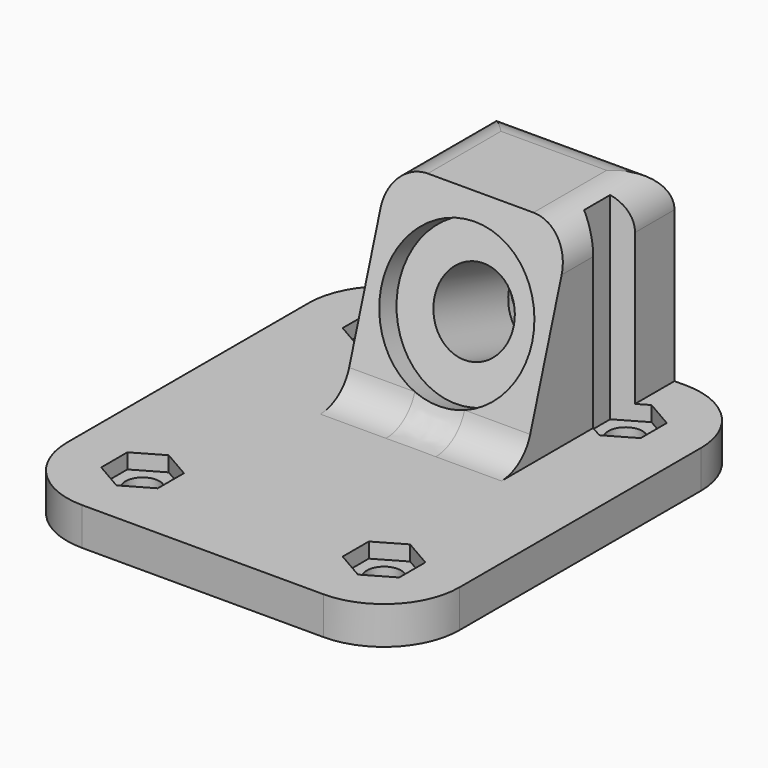
from build123d import *

# Parameters (mm, degrees)
F0_W         = 52
F0_H         = 60
F1_DEPTH     = 5
F2_R         = 10
F3_R         = 2.25
F4_DEPTH     = 25
F6_DEPTH     = 2
F7_W         = 24
F7_H         = 25
F8_DEPTH     = 25
F10_DEPTH    = 35.501
F11_R        = 5.25
F12_DEPTH    = 25.3474527662
F13_R        = 10
F13_R_2      = 5.25
F14_DEPTH    = 3
F16_R        = 10
F17_DEPTH    = 12
F18_DEPTH    = 25.001
F19_F1_R     = 5
F19_T2_DEPTH = 42.117530278
F19_T4_DEPTH = 31.5358983849
F19_T6_DEPTH = 28.6534286629
F19_T8_DEPTH = 49


# Not quite as in the source:
# - a fillet or chamfer that OpenCascade refuses, or shapes differently, is made with other operations: its cross-section is extruded or revolved along the edge and cut away or added


with BuildPart() as f1:
    # F0 (on Top) → F1 (new body)
    with BuildSketch(Plane.XY):
        Rectangle(F0_W, F0_H)
    extrude(amount=F1_DEPTH)

    # F2
    f2_edges = [f1.edges().sort_by_distance(p)[0] for p in [
        (26, -30, 2.5),
        (-26, -30, 2.5),
        (26, 30, 2.5),
        (-26, 30, 2.5),
    ]]
    fillet(f2_edges, radius=F2_R)

    # F3 (on face) → F4 (cut)
    with BuildSketch(Plane.XY.offset(5)):
        with Locations((-16, -20)):
            Circle(F3_R)
        with Locations((16, -20)):
            Circle(F3_R)
        with Locations((-16, 20)):
            Circle(F3_R)
        with Locations((16, 20)):
            Circle(F3_R)
    extrude(amount=-F4_DEPTH, mode=Mode.SUBTRACT)

    # F5 (on face) → F6 (cut)
    with BuildSketch(Plane.XY.offset(5)):
        Polygon((-16, -15.6698729811), (-19.75, -17.8349364905), (-19.75, -22.1650635095), (-16, -24.3301270189), (-12.25, -22.1650635095), (-12.25, -17.8349364905), align=None)
        Polygon((-12.25, 22.1650635095), (-16, 24.3301270189), (-19.75, 22.1650635095), (-19.75, 17.8349364905), (-16, 15.6698729811), (-12.25, 17.8349364905), align=None)
        Polygon((19.75, -17.8349364905), (16, -15.6698729811), (12.25, -17.8349364905), (12.25, -22.1650635095), (16, -24.3301270189), (19.75, -22.1650635095), align=None)
        Polygon((19.75, 22.1650635095), (16, 24.3301270189), (12.25, 22.1650635095), (12.25, 17.8349364905), (16, 15.6698729811), (19.75, 17.8349364905), align=None)
    extrude(amount=-F6_DEPTH, mode=Mode.SUBTRACT)

    # F7 (on face) → F8 (join)
    with BuildSketch(Plane.XY.offset(5)):
        with Locations((2.5, 17.5)):
            Rectangle(F7_W, F7_H)
    extrude(amount=F8_DEPTH)

    # F9 (on face) → F10 (cut, through all)
    with BuildSketch(Plane(origin=(-9.5, 0, 0), x_dir=(0, -1, 0), z_dir=(-1, 0, 0))):
        Polygon((-12.882469722, 30), (-5, 5), (-5, 30), align=None)
    extrude(amount=-F10_DEPTH, mode=Mode.SUBTRACT)

    # F11 (on face) → F12 (cut, through all)
    with BuildSketch(Plane(origin=(0, 3.1139390198, -0.9818212016), x_dir=(1, 0, 0), z_dir=(0, -0.9537169507, 0.3007057995))):
        with Locations((2.5, 19.3787278155)):
            Circle(F11_R)
    extrude(amount=-F12_DEPTH, mode=Mode.SUBTRACT)

    # F13 (on face) → F14 (cut)
    with BuildSketch(Plane(origin=(0, 3.1139390198, -0.9818212016), x_dir=(1, 0, 0), z_dir=(0, -0.9537169507, 0.3007057995))):
        with Locations((2.5, 19.3787278155)):
            Circle(F13_R)
        with Locations((2.5, 19.3787278155)):
            Circle(F13_R_2, mode=Mode.SUBTRACT)
    extrude(amount=-F14_DEPTH, mode=Mode.SUBTRACT)

    # F16 (on offset) → F17 (cut)
    with BuildSketch(Plane(origin=(0, 29.8180136408, -9.4015835877), x_dir=(1, 0, 0), z_dir=(0, -0.9537169507, 0.3007057995))):
        with Locations((2.5, 19.3787278155)):
            Circle(F16_R)
    extrude(amount=F17_DEPTH, mode=Mode.SUBTRACT)

    # F5 (on face) → F18 (cut, through all)
    with BuildSketch(Plane.XY.offset(5)):
        Polygon((-16, -15.6698729811), (-19.75, -17.8349364905), (-19.75, -22.1650635095), (-16, -24.3301270189), (-12.25, -22.1650635095), (-12.25, -17.8349364905), align=None)
        Polygon((-12.25, 22.1650635095), (-16, 24.3301270189), (-19.75, 22.1650635095), (-19.75, 17.8349364905), (-16, 15.6698729811), (-12.25, 17.8349364905), align=None)
        Polygon((19.75, -17.8349364905), (16, -15.6698729811), (12.25, -17.8349364905), (12.25, -22.1650635095), (16, -24.3301270189), (19.75, -22.1650635095), align=None)
        Polygon((19.75, 22.1650635095), (16, 24.3301270189), (12.25, 22.1650635095), (12.25, 17.8349364905), (16, 15.6698729811), (19.75, 17.8349364905), align=None)
    extrude(amount=F18_DEPTH, mode=Mode.SUBTRACT)

    # F19: fillet of radius 5 on 5 edges, made by hand

    # F19_f1
    f19_f1_edges = [f1.edges().sort_by_distance(p)[0] for p in [
        (2.5, 5, 5),
    ]]
    fillet(f19_f1_edges, radius=F19_F1_R)

    # F19_s3 → F19_t2 (cut)
    with BuildSketch(Plane.XZ.offset(-42.5)):
        with BuildLine():
            ThreePointArc((-9.5, 25), (-8.0355339059, 28.5355339059), (-4.5, 30))
            Line((-4.5, 30), (-4.5, 30.1))
            Line((-4.5, 30.1), (-9.6, 30.1))
            Line((-9.6, 30.1), (-9.6, 25))
            Line((-9.6, 25), (-9.5, 25))
        make_face()
    extrude(amount=F19_T2_DEPTH, mode=Mode.SUBTRACT)

    # F19_s5 → F19_t4 (cut)
    with BuildSketch(Plane.XZ.offset(-42.5)):
        with BuildLine():
            ThreePointArc((14.5, 25), (13.0355339059, 28.5355339059), (9.5, 30))
            Line((9.5, 30), (9.5, 30.1))
            Line((9.5, 30.1), (14.6, 30.1))
            Line((14.6, 30.1), (14.6, 25))
            Line((14.6, 25), (14.5, 25))
        make_face()
    extrude(amount=F19_T4_DEPTH, mode=Mode.SUBTRACT)

    # F19_s7 → F19_t6 (cut)
    with BuildSketch(Plane.XZ.offset(-29.0358983849)):
        with BuildLine():
            ThreePointArc((14.5, 25), (13.0355339059, 28.5355339059), (9.5, 30))
            Line((9.5, 30), (9.5, 30.1))
            Line((9.5, 30.1), (14.6, 30.1))
            Line((14.6, 30.1), (14.6, 25))
            Line((14.6, 25), (14.5, 25))
        make_face()
    extrude(amount=F19_T6_DEPTH, mode=Mode.SUBTRACT)

    # F19_s9 → F19_t8 (cut)
    with BuildSketch(Plane.YZ.offset(-22)):
        with BuildLine():
            ThreePointArc((30, 25), (28.5355339059, 28.5355339059), (25, 30))
            Line((25, 30), (25, 30.1))
            Line((25, 30.1), (30.1, 30.1))
            Line((30.1, 30.1), (30.1, 25))
            Line((30.1, 25), (30, 25))
        make_face()
    extrude(amount=F19_T8_DEPTH, mode=Mode.SUBTRACT)


solid = f1.part
